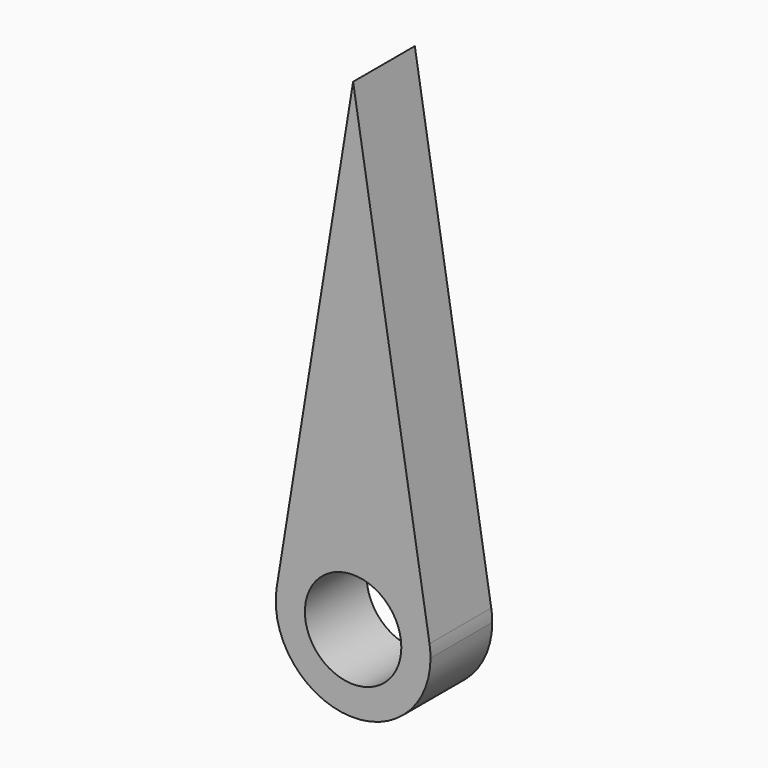
from build123d import *

# Parameters (mm, degrees)
F0_R     = 1.5875
F1_DEPTH = 1.27
F2_DEPTH = 1.27


with BuildPart() as f1:
    # F0 (on Front) → F1 (new body, symmetric)
    with BuildSketch(Plane.XZ):
        with BuildLine():
            ThreePointArc((-2.514835, 0.40892), (-0.205126, -2.539593), (2.547864, 0))
            ThreePointArc((2.547864, 0), (2.539593, 0.205126), (2.514835, 0.40892))
            ThreePointArc((2.514835, 0.40892), (0, 2.547864), (-2.514835, 0.40892))
        make_face()
        Circle(F0_R, mode=Mode.SUBTRACT)
    extrude(amount=F1_DEPTH, both=True)

    # F0 (on Front) → F2 (join, symmetric)
    with BuildSketch(Plane.XZ):
        with BuildLine():
            ThreePointArc((-2.514835, 0.40892), (0, 2.547864), (2.514835, 0.40892))
            Line((2.514835, 0.40892), (0, 15.875))
            Line((0, 15.875), (-2.514835, 0.40892))
        make_face()
    extrude(amount=F2_DEPTH, both=True)


solid = f1.part
